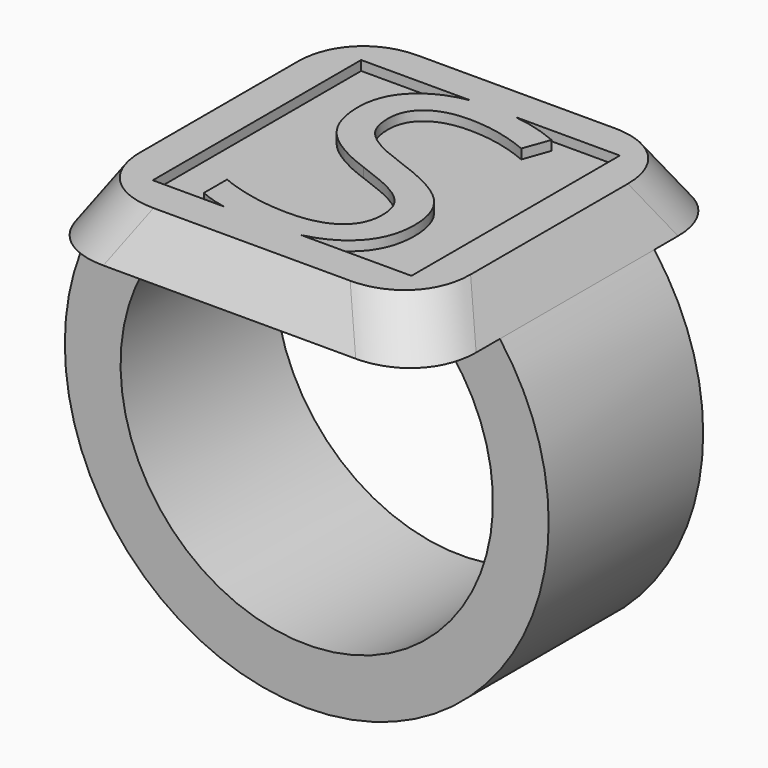
from build123d import *

# Parameters (mm, degrees)
F0_W          = 25.4
F0_H          = 25.4
F1_DEPTH      = 3.175
F1_TAPER      = 30
F3_W          = 5.08
F3_H          = 12.7
F7_DEPTH      = 6.35
F8_R          = 5.08
F9_W          = 17.0137826353
F9_H          = 17.1311190352
F10_DEPTH     = 0.635
F11_TEXT_SIZE = 23.7932208822
F12_DEPTH     = 0.635
F13_SCALE     = 0.83


# Not quite as in the source:
# - a feature names something its author has since deleted; it is built from what else it names
# - Text() gives the source's letters only with a copy of the font that has no kerning and outlines rounded to 1/6400 em; it was checked with that copy


with BuildPart() as f1:
    # F0 (on Top) → F1 (new body)
    with BuildSketch(Plane.XY):
        Rectangle(F0_W, F0_H)
    extrude(amount=F1_DEPTH, taper=F1_TAPER)

    # F4: sweep along a path in F2
    with BuildLine(Plane.XZ) as f4_path:
        ThreePointArc((-10.16, 0), (0, -23.5582897328), (10.16, 0))
    # F3 (on face) → F4 (sweep)
    with BuildSketch(Plane(origin=(0, 0, 0), x_dir=(1, 0, 0), z_dir=(0, 0, -1))):
        with Locations((10.16, 0)):
            Rectangle(F3_W, F3_H)
    sweep(path=f4_path.line)

    # F6 (on Front) → F7 (join, symmetric)
    with BuildSketch(Plane.XZ):
        with BuildLine():
            Line((-7.62, 0), (-10.16, 0))
            Line((-10.16, 0), (-10.0130578512, -2.535746045))
            ThreePointArc((-10.0130578512, -2.535746045), (-8.9072265211, -1.1822790439), (-7.62, 0))
        make_face()
    extrude(amount=F7_DEPTH, both=True)

    # F8
    f8_edges = [f1.edges().sort_by_distance(p)[0] for p in [
        (-11.783456, 11.783456, 1.5875),
        (11.783456, 11.783456, 1.5875),
        (11.783456, -11.783456, 1.5875),
        (-11.783456, -11.783456, 1.5875),
    ]]
    fillet(f8_edges, radius=F8_R)

    # F9 (on face) → F10 (cut, symmetric)
    with BuildSketch(Plane.XY.offset(3.175)):
        with Locations((0.0785226002, 0.0907643698)):
            Rectangle(F9_W, F9_H)
    extrude(amount=F10_DEPTH, both=True, mode=Mode.SUBTRACT)

    # F11 (on face) → F12 (join)
    with BuildSketch(Plane.XY.offset(2.54)):
        with Locations((-6.7308791261, -8.4747951478)):
            Text('S', F11_TEXT_SIZE, font='Open Sans', text_align=(TextAlign.LEFT, TextAlign.BOTTOM))
    extrude(amount=F12_DEPTH)


with BuildPart() as f1_1:
    # F13: moved
    add(f1.part.scale(F13_SCALE))


solid = f1_1.part
